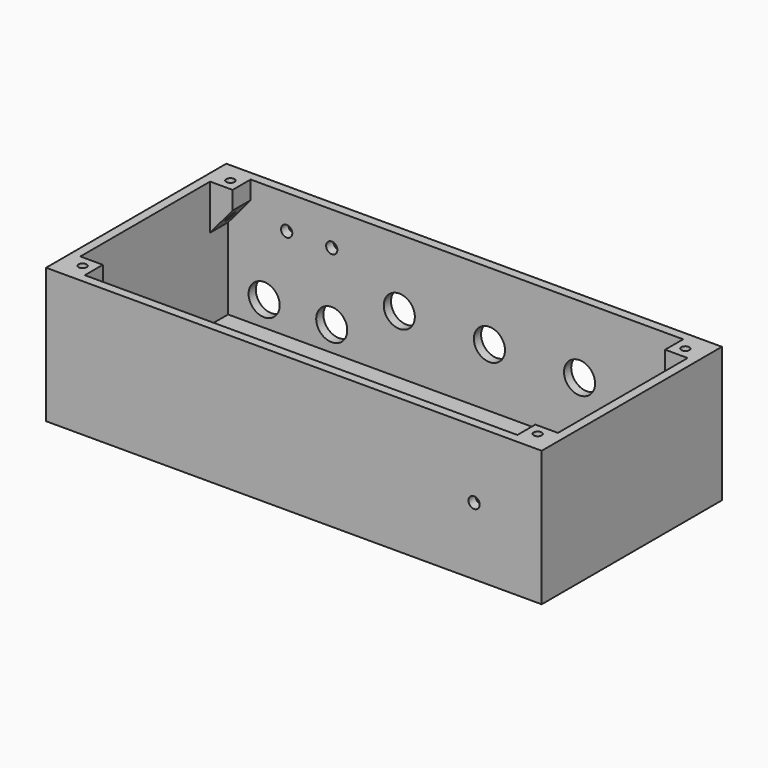
from build123d import *

# Parameters (mm, degrees)
F0_W        = 139.7
F0_H        = 63.5
F1_DEPTH    = 19.05
F2_W        = 134.62
F2_H        = 58.42
F3_DEPTH    = 35.56
F4_R        = 1.5875
F5_DEPTH    = 2.54
F6_R        = 4.3815
F6_R_2      = 1.5875
F7_DEPTH    = 2.54
F8_W        = 6.35
F8_H        = 6.35
F9_DEPTH    = 12.7
F10_SIZE2   = 7.567625
F10_SIZE    = 6.34999
F10_2_SIZE2 = 7.567625
F10_2_SIZE  = 6.34999
F11_SIZE2   = 7.567625
F11_SIZE    = 6.34999
F11_2_SIZE2 = 7.567625
F11_2_SIZE  = 6.34999
F12_R       = 1.143
F13_DEPTH   = 12.7


# Not quite as in the source:
# - a fillet or chamfer is up to 0.001 mm smaller than in the source, because OpenCascade refuses the exact size


with BuildPart() as f1:
    # F0 (on Top) → F1 (new body, symmetric)
    with BuildSketch(Plane.XY):
        Rectangle(F0_W, F0_H)
    extrude(amount=F1_DEPTH, both=True)

    # F2 (on face) → F3 (cut)
    with BuildSketch(Plane.XY.offset(19.05)):
        Rectangle(F2_W, F2_H)
    extrude(amount=-F3_DEPTH, mode=Mode.SUBTRACT)

    # F4 (on face) → F5 (cut, through all)
    with BuildSketch(Plane.XZ.offset(31.75)):
        with Locations((50.8, 0)):
            Circle(F4_R)
    extrude(amount=-F5_DEPTH, mode=Mode.SUBTRACT)

    # F6 (on face) → F7 (cut, through all)
    with BuildSketch(Plane(origin=(0, 31.75, 0), x_dir=(-1, 0, 0), z_dir=(0, 1, 0))):
        with Locations((-31.75, 0)):
            Circle(F6_R)
        with Locations((-6.35, 0)):
            Circle(F6_R)
        with Locations((19.05, 0)):
            Circle(F6_R)
        with Locations((50.8, 9.525)):
            Circle(F6_R_2)
        with Locations((38.1, 9.525)):
            Circle(F6_R_2)
        with Locations((57.15, -9.525)):
            Circle(F6_R)
        with Locations((38.1, -9.525)):
            Circle(F6_R)
        with Locations((-57.15, 0)):
            Circle(F6_R)
    extrude(amount=-F7_DEPTH, mode=Mode.SUBTRACT)

    # F8 (on face) → F9 (join)
    with BuildSketch(Plane.XY.offset(19.05)):
        with Locations((-64.135, -26.035)):
            Rectangle(F8_W, F8_H)
        with Locations((64.135, 26.035)):
            Rectangle(F8_W, F8_H)
        with Locations((64.135, -26.035)):
            Rectangle(F8_W, F8_H)
        with Locations((-64.135, 26.035)):
            Rectangle(F8_W, F8_H)
    extrude(amount=-F9_DEPTH)

    # F10 (size 6.35 and 7.567635313 in the source; OpenCascade refuses exactly that, so slightly less here)
    f10_edges = [f1.edges().sort_by_distance(p)[0] for p in [
        (-60.96, 26.035, 6.35),
    ]]
    f10_side = f1.faces().sort_by_distance((-64.135, 26.035, 6.35))[0]
    chamfer(f10_edges, length=F10_SIZE, length2=F10_SIZE2, reference=f10_side)

    # F10#2 (size 6.35 and 7.567635313 in the source; OpenCascade refuses exactly that, so slightly less here)
    f10_2_edges = [f1.edges().sort_by_distance(p)[0] for p in [
        (60.96, -26.035, 6.35),
    ]]
    f10_2_side = f1.faces().sort_by_distance((64.135, -26.035, 6.35))[0]
    chamfer(f10_2_edges, length=F10_2_SIZE, length2=F10_2_SIZE2, reference=f10_2_side)

    # F11 (size 6.35 and 7.567635313 in the source; OpenCascade refuses exactly that, so slightly less here)
    f11_edges = [f1.edges().sort_by_distance(p)[0] for p in [
        (60.96, 26.035, 6.35),
    ]]
    f11_side = f1.faces().sort_by_distance((64.135, 26.035, 6.35))[0]
    chamfer(f11_edges, length=F11_SIZE, length2=F11_SIZE2, reference=f11_side)

    # F11#2 (size 6.35 and 7.567635313 in the source; OpenCascade refuses exactly that, so slightly less here)
    f11_2_edges = [f1.edges().sort_by_distance(p)[0] for p in [
        (-60.96, -26.035, 6.35),
    ]]
    f11_2_side = f1.faces().sort_by_distance((-64.135, -26.035, 6.35))[0]
    chamfer(f11_2_edges, length=F11_2_SIZE, length2=F11_2_SIZE2, reference=f11_2_side)

    # F12 (on face) → F13 (cut)
    with BuildSketch(Plane.XY.offset(19.05)):
        with Locations((-64.135, 26.035)):
            Circle(F12_R)
        with Locations((64.135, 26.035)):
            Circle(F12_R)
        with Locations((-64.135, -26.035)):
            Circle(F12_R)
        with Locations((64.135, -26.035)):
            Circle(F12_R)
    extrude(amount=-F13_DEPTH, mode=Mode.SUBTRACT)


solid = f1.part
